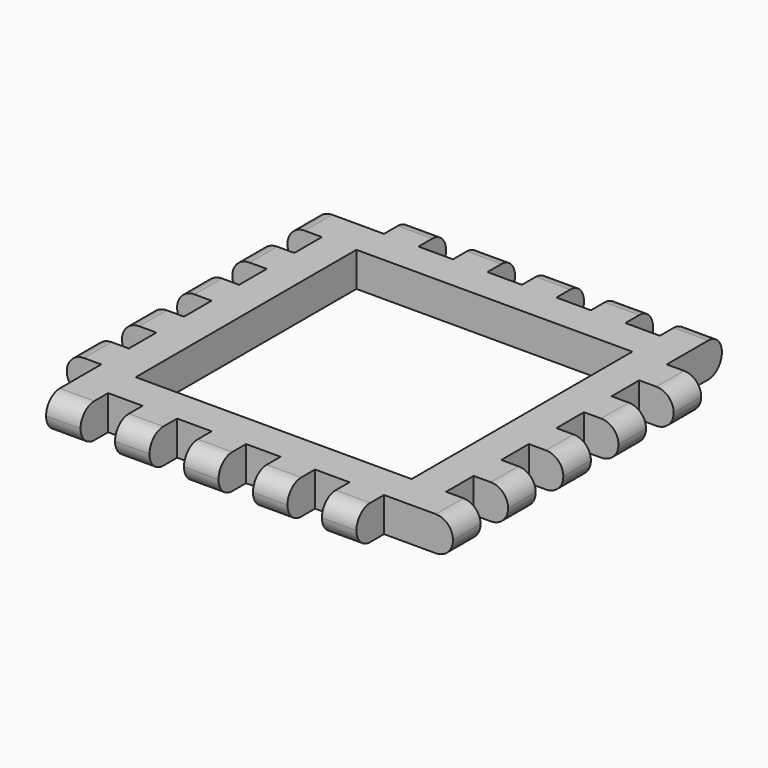
from build123d import *

# Parameters (mm, degrees)
F0_W     = 40
F0_H     = 40
F0_W_2   = 5
F0_H_2   = 5
F1_DEPTH = 5
F2_R     = 2.49999


# Not quite as in the source:
# - a fillet or chamfer is up to 0.001 mm smaller than in the source, because OpenCascade refuses the exact size


with BuildPart() as f1:
    # F0 (on Top) → F1 (new body)
    with BuildSketch(Plane.XY):
        Polygon((25, 20), (25, 25), (20, 25), (15, 25), (10, 25), (5, 25), (0, 25), (-5, 25), (-10, 25), (-15, 25), (-20, 25), (-25, 25), (-25, 20), (-25, 15), (-25, 10), (-25, 5), (-25, 0), (-25, -5), (-25, -10), (-25, -15), (-25, -20), (-25, -25), (-20, -25), (-15, -25), (-10, -25), (-5, -25), (0, -25), (5, -25), (10, -25), (15, -25), (20, -25), (25, -25), (25, -20), (25, -15), (25, -10), (25, -5), (25, 0), (25, 5), (25, 10), (25, 15), align=None)
        Rectangle(F0_W, F0_H, mode=Mode.SUBTRACT)
        with Locations((22.5, 27.5)):
            Rectangle(F0_W_2, F0_H_2)
        with Locations((27.5, 17.5)):
            Rectangle(F0_W_2, F0_H_2)
        with Locations((12.5, 27.5)):
            Rectangle(F0_W_2, F0_H_2)
        with Locations((27.5, 7.5)):
            Rectangle(F0_W_2, F0_H_2)
        with Locations((2.5, 27.5)):
            Rectangle(F0_W_2, F0_H_2)
        with Locations((27.5, -2.5)):
            Rectangle(F0_W_2, F0_H_2)
        with Locations((-7.5, 27.5)):
            Rectangle(F0_W_2, F0_H_2)
        with Locations((27.5, -12.5)):
            Rectangle(F0_W_2, F0_H_2)
        with Locations((-17.5, 27.5)):
            Rectangle(F0_W_2, F0_H_2)
        with Locations((27.5, -22.5)):
            Rectangle(F0_W_2, F0_H_2)
        with Locations((-27.5, 22.5)):
            Rectangle(F0_W_2, F0_H_2)
        with Locations((17.5, -27.5)):
            Rectangle(F0_W_2, F0_H_2)
        with Locations((-27.5, 12.5)):
            Rectangle(F0_W_2, F0_H_2)
        with Locations((7.5, -27.5)):
            Rectangle(F0_W_2, F0_H_2)
        with Locations((-27.5, 2.5)):
            Rectangle(F0_W_2, F0_H_2)
        with Locations((-2.5, -27.5)):
            Rectangle(F0_W_2, F0_H_2)
        with Locations((-27.5, -7.5)):
            Rectangle(F0_W_2, F0_H_2)
        with Locations((-12.5, -27.5)):
            Rectangle(F0_W_2, F0_H_2)
        with Locations((-27.5, -17.5)):
            Rectangle(F0_W_2, F0_H_2)
        with Locations((-22.5, -27.5)):
            Rectangle(F0_W_2, F0_H_2)
    extrude(amount=F1_DEPTH)

    # F2 (radius 2.5 in the source; OpenCascade refuses exactly that, so slightly less here)
    f2_edges = [f1.edges().sort_by_distance(p)[0] for p in [
        (-30, 22.5, 5),
        (-30, 22.5, 0),
        (-30, 12.5, 5),
        (-30, 12.5, 0),
        (-30, 2.5, 0),
        (-30, 2.5, 5),
        (-30, -7.5, 0),
        (-30, -7.5, 5),
        (-30, -17.5, 5),
        (-30, -17.5, 0),
        (-22.5, -30, 5),
        (-22.5, -30, 0),
        (-12.5, -30, 5),
        (-12.5, -30, 0),
        (-2.5, -30, 0),
        (-2.5, -30, 5),
        (7.5, -30, 5),
        (7.5, -30, 0),
        (17.5, -30, 0),
        (17.5, -30, 5),
        (30, -22.5, 5),
        (30, -22.5, 0),
        (30, -12.5, 5),
        (30, -12.5, 0),
        (30, -2.5, 5),
        (30, -2.5, 0),
        (30, 7.5, 5),
        (30, 7.5, 0),
        (30, 17.5, 5),
        (30, 17.5, 0),
        (22.5, 30, 5),
        (22.5, 30, 0),
        (12.5, 30, 5),
        (2.5, 30, 5),
        (2.5, 30, 0),
        (-7.5, 30, 5),
        (-7.5, 30, 0),
        (-17.5, 30, 5),
        (-17.5, 30, 0),
    ]]
    fillet(f2_edges, radius=F2_R)


solid = f1.part
